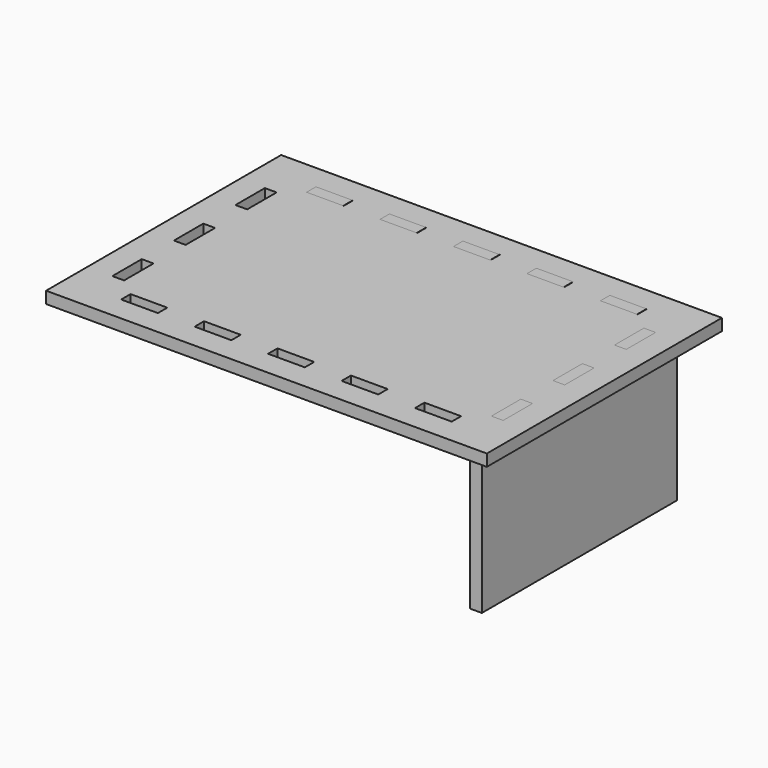
from build123d import *

# Parameters (mm, degrees)
F1_W     = 152.4
F1_H     = 101.6
F1_W_2   = 12.7
F1_H_2   = 4.064
F1_W_3   = 4.064
F1_H_3   = 12.7
F2_DEPTH = 4.064
F3_W     = 12.7
F3_H     = 4.064
F4_DEPTH = 4.064
F5_W     = 12.7
F5_H     = 4.064
F6_DEPTH = 4.064


with BuildPart() as f2:
    # F1 (on Top) → F2 (new body)
    with BuildSketch(Plane.XY):
        with Locations((76.2, -50.8)):
            Rectangle(F1_W, F1_H)
        with Locations((25.4, -90.932)):
            Rectangle(F1_W_2, F1_H_2, mode=Mode.SUBTRACT)
        with Locations((10.668, -77.3989244119)):
            Rectangle(F1_W_3, F1_H_3, mode=Mode.SUBTRACT)
        with Locations((50.8, -90.932)):
            Rectangle(F1_W_2, F1_H_2, mode=Mode.SUBTRACT)
        with Locations((76.2, -90.932)):
            Rectangle(F1_W_2, F1_H_2, mode=Mode.SUBTRACT)
        with Locations((10.668, -50.8)):
            Rectangle(F1_W_3, F1_H_3, mode=Mode.SUBTRACT)
        with Locations((101.6, -90.932)):
            Rectangle(F1_W_2, F1_H_2, mode=Mode.SUBTRACT)
        with Locations((127, -90.932)):
            Rectangle(F1_W_2, F1_H_2, mode=Mode.SUBTRACT)
        with Locations((141.732, -77.3989244119)):
            Rectangle(F1_W_3, F1_H_3, mode=Mode.SUBTRACT)
        with Locations((141.732, -50.8)):
            Rectangle(F1_W_3, F1_H_3, mode=Mode.SUBTRACT)
        with Locations((10.668, -24.2010755881)):
            Rectangle(F1_W_3, F1_H_3, mode=Mode.SUBTRACT)
        with Locations((25.4, -10.668)):
            Rectangle(F1_W_2, F1_H_2, mode=Mode.SUBTRACT)
        with Locations((50.8, -10.668)):
            Rectangle(F1_W_2, F1_H_2, mode=Mode.SUBTRACT)
        with Locations((76.2, -10.668)):
            Rectangle(F1_W_2, F1_H_2, mode=Mode.SUBTRACT)
        with Locations((101.6, -10.668)):
            Rectangle(F1_W_2, F1_H_2, mode=Mode.SUBTRACT)
        with Locations((141.732, -24.2010755881)):
            Rectangle(F1_W_3, F1_H_3, mode=Mode.SUBTRACT)
        with Locations((127, -10.668)):
            Rectangle(F1_W_2, F1_H_2, mode=Mode.SUBTRACT)
    extrude(amount=F2_DEPTH)


with BuildPart() as f4:
    # F3 (on face) → F4 (new body)
    with BuildSketch(Plane(origin=(0, -12.7, 0), x_dir=(-1, 0, 0), z_dir=(0, 1, 0))):
        Polygon((-12.6052666744, -50.8), (-12.6052666744, 0), (-18.9552666744, 0), (-31.6552666744, 0), (-44.3552666744, 0), (-57.0552666744, 0), (-69.7552666744, 0), (-82.4552666744, 0), (-95.1552666744, 0), (-107.8552666744, 0), (-120.5552666744, 0), (-133.2552666744, 0), (-139.6052666744, 0), (-139.6052666744, -50.8), align=None)
        with Locations((-25.3052666744, 2.032)):
            Rectangle(F3_W, F3_H)
        with Locations((-50.7052666744, 2.032)):
            Rectangle(F3_W, F3_H)
        with Locations((-126.9052666744, 2.032)):
            Rectangle(F3_W, F3_H)
        with Locations((-76.1052666744, 2.032)):
            Rectangle(F3_W, F3_H)
        with Locations((-101.5052666744, 2.032)):
            Rectangle(F3_W, F3_H)
    extrude(amount=F4_DEPTH)


with BuildPart() as f6:
    # F5 (on face) → F6 (new body)
    with BuildSketch(Plane.YZ.offset(139.7)):
        with Locations((-50.8, 2.032)):
            Rectangle(F5_W, F5_H)
        with Locations((-24.2010755881, 2.032)):
            Rectangle(F5_W, F5_H)
        with Locations((-77.3989244119, 2.032)):
            Rectangle(F5_W, F5_H)
        Polygon((-8.636, -50.8), (-8.636, 0), (-17.8510755881, 0), (-30.5510755881, 0), (-44.45, 0), (-57.15, 0), (-71.0489244119, 0), (-83.7489244119, 0), (-92.964, 0), (-92.964, -50.8), align=None)
    extrude(amount=F6_DEPTH)


solid = Compound([f2.part, f4.part, f6.part])
